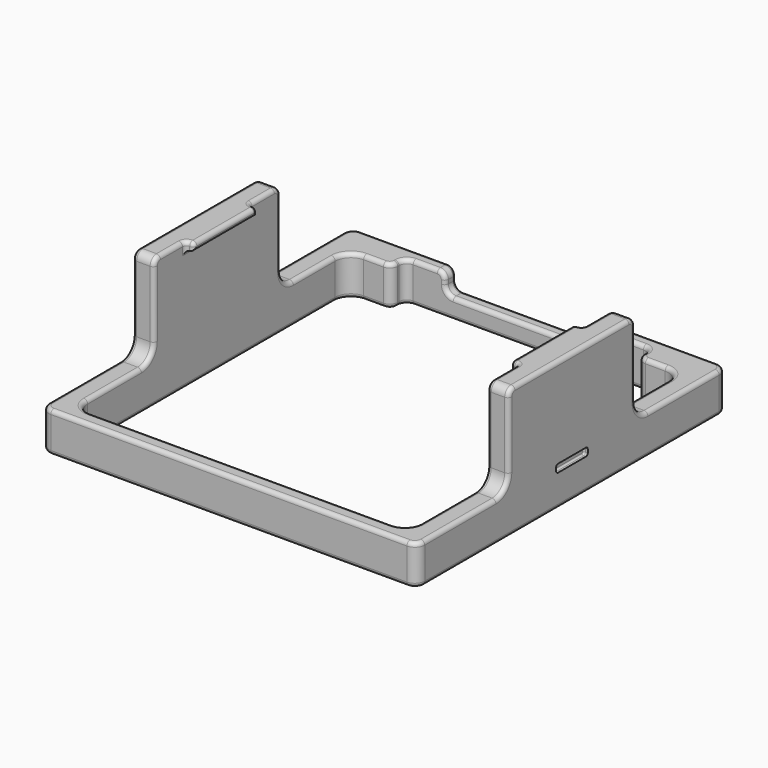
from build123d import *

# Parameters (mm, degrees)
F1_DEPTH      = 12.7
F2_W          = 53.34
F2_H          = 6.35
F3_DEPTH      = 4.318
F4_W          = 6.858
F4_H          = 50.8
F5_DEPTH      = 28.956
F7_W          = 25.4
F7_H          = 2.54
F8_DEPTH      = 2.54
F6_W          = 25.4
F6_H          = 2.54
F9_DEPTH      = 2.54
F10_R         = 5.08
F11_R         = 2.54
F12_R         = 1.26999
F13_R         = 2.54
F14_R         = 1.26999
F15_R         = 1.27
F16_W         = 12.7
F16_H         = 2.54
F18_DEPTH     = 1.27
F17_W         = 12.7
F17_H         = 2.54
F19_DEPTH     = 1.27
F20_R         = 0.508
F21_T1_DEPTH  = 1.27
F21_T3_DEPTH  = 1.27
F21_T6_ANGLE  = 90
F21_T8_ANGLE  = 90
F21_T10_ANGLE = 90
F21_T12_ANGLE = 90
F21_T14_ANGLE = 90
F21_T16_ANGLE = 90
F21_T18_ANGLE = 90
F21_T20_ANGLE = 90


# Not quite as in the source:
# - a fillet or chamfer that OpenCascade refuses, or shapes differently, is made with other operations: its cross-section is extruded or revolved along the edge and cut away or added
# - a fillet or chamfer is up to 0.001 mm smaller than in the source, because OpenCascade refuses the exact size


with BuildPart() as f1:
    # F0 (on Top) → F1 (new body)
    with BuildSketch(Plane.XY):
        with BuildLine():
            ThreePointArc((-60.325, -59.055), (-59.3950640303, -61.3000640303), (-57.15, -62.23))
            Line((-57.15, -62.23), (57.15, -62.23))
            ThreePointArc((57.15, -62.23), (59.3950640303, -61.3000640303), (60.325, -59.055))
            Line((60.325, -59.055), (60.325, 59.055))
            ThreePointArc((60.325, 59.055), (59.3950640303, 61.3000640303), (57.15, 62.23))
            Line((57.15, 62.23), (-57.15, 62.23))
            ThreePointArc((-57.15, 62.23), (-59.3950640303, 61.3000640303), (-60.325, 59.055))
            Line((-60.325, 59.055), (-60.325, -59.055))
        make_face()
        with BuildLine():
            Line((39.497, 52.324), (48.387, 52.324))
            ThreePointArc((48.387, 52.324), (51.9791024484, 50.8361024484), (53.467, 47.244))
            Line((53.467, 47.244), (53.467, -52.07))
            ThreePointArc((53.467, -52.07), (51.9791024484, -55.6621024484), (48.387, -57.15))
            Line((48.387, -57.15), (-48.387, -57.15))
            ThreePointArc((-48.387, -57.15), (-51.9791024484, -55.6621024484), (-53.467, -52.07))
            Line((-53.467, -52.07), (-53.467, 47.244))
            ThreePointArc((-53.467, 47.244), (-51.9791024484, 50.8361024484), (-48.387, 52.324))
            Line((-48.387, 52.324), (-39.497, 52.324))
            Line((-39.497, 52.324), (-39.497, 57.912))
            Line((-39.497, 57.912), (39.497, 57.912))
            Line((39.497, 57.912), (39.497, 52.324))
        make_face(mode=Mode.SUBTRACT)
    extrude(amount=F1_DEPTH)

    # F2 (on face) → F3 (cut, through all)
    with BuildSketch(Plane(origin=(0, 62.23, 0), x_dir=(-1, 0, 0), z_dir=(0, 1, 0))):
        with Locations((0, 9.525)):
            Rectangle(F2_W, F2_H)
    extrude(amount=-F3_DEPTH, mode=Mode.SUBTRACT)

    # F4 (on face) → F5 (join)
    with BuildSketch(Plane.XY.offset(12.7)):
        with Locations((56.896, 0)):
            Rectangle(F4_W, F4_H)
        with Locations((-56.896, 0)):
            Rectangle(F4_W, F4_H)
    extrude(amount=F5_DEPTH)

    # F7 (on face) → F8 (join)
    with BuildSketch(Plane(origin=(53.467, 0, 0), x_dir=(0, -1, 0), z_dir=(-1, 0, 0))):
        with Locations((0, 40.386)):
            Rectangle(F7_W, F7_H)
    extrude(amount=F8_DEPTH)

    # F6 (on face) → F9 (join)
    with BuildSketch(Plane.YZ.offset(-53.467)):
        with Locations((0, 40.386)):
            Rectangle(F6_W, F6_H)
    extrude(amount=F9_DEPTH)

    # F10
    f10_edges = [f1.edges().sort_by_distance(p)[0] for p in [
        (56.896, 25.4, 12.7),
        (-56.896, 25.4, 12.7),
        (56.896, -25.4, 12.7),
        (-56.896, -25.4, 12.7),
    ]]
    fillet(f10_edges, radius=F10_R)

    # F11
    f11_edges = [f1.edges().sort_by_distance(p)[0] for p in [
        (-56.896, -25.4, 41.656),
        (-56.896, 25.4, 41.656),
        (56.896, -25.4, 41.656),
        (56.896, 25.4, 41.656),
    ]]
    fillet(f11_edges, radius=F11_R)

    # F12 (radius 1.27 in the source; OpenCascade refuses exactly that, so slightly less here)
    f12_edges = [f1.edges().sort_by_distance(p)[0] for p in [
        (-50.927, -12.7, 40.386),
        (-50.927, 12.7, 40.386),
        (50.927, 12.7, 40.386),
        (50.927, -12.7, 40.386),
        (53.467, 0, 39.116),
        (-53.467, 0, 39.116),
        (-53.467, 12.7, 40.386),
        (53.467, 12.7, 40.386),
        (53.467, -12.7, 40.386),
        (-53.467, -12.7, 40.386),
        (50.927, 0, 39.116),
        (-50.927, 0, 39.116),
    ]]
    fillet(f12_edges, radius=F12_R)

    # F13
    f13_edges = [f1.edges().sort_by_distance(p)[0] for p in [
        (-39.497, 52.324, 6.35),
        (-26.67, 60.071, 12.7),
        (26.67, 60.071, 12.7),
        (39.497, 52.324, 6.35),
        (-39.497, 57.912, 6.35),
        (39.497, 57.912, 6.35),
        (26.67, 60.071, 6.35),
        (-26.67, 60.071, 6.35),
    ]]
    fillet(f13_edges, radius=F13_R)

    # F14 (radius 1.27 in the source; OpenCascade refuses exactly that, so slightly less here)
    f14_edges = [f1.edges().sort_by_distance(p)[0] for p in [
        (-53.467, 38.862, 12.7),
        (-51.979102, 50.836102, 12.7),
        (60.325, 44.7675, 12.7),
        (-43.18, 62.23, 12.7),
        (43.18, 62.23, 12.7),
        (59.395064, 61.300064, 12.7),
        (-59.395064, 61.300064, 12.7),
        (-60.325, 44.7675, 12.7),
        (60.325, 0, 0),
        (59.395064, 61.300064, 0),
    ]]
    fillet(f14_edges, radius=F14_R)

    # F15
    f15_edges = [f1.edges().sort_by_distance(p)[0] for p in [
        (-45.212, 52.324, 0),
        (-40.240949, 53.067949, 0),
    ]]
    fillet(f15_edges, radius=F15_R)

    # F16 (on face) → F18 (cut)
    with BuildSketch(Plane(origin=(-60.325, 0, 0), x_dir=(0, -1, 0), z_dir=(-1, 0, 0))):
        with Locations((0, 11.43)):
            Rectangle(F16_W, F16_H)
    extrude(amount=-F18_DEPTH, mode=Mode.SUBTRACT)

    # F17 (on face) → F19 (cut)
    with BuildSketch(Plane.YZ.offset(60.325)):
        with Locations((0, 11.43)):
            Rectangle(F17_W, F17_H)
    extrude(amount=-F19_DEPTH, mode=Mode.SUBTRACT)

    # F20
    f20_edges = [f1.edges().sort_by_distance(p)[0] for p in [
        (-59.055, 0, 10.16),
        (-59.055, 6.35, 11.43),
        (-59.055, 0, 12.7),
        (-59.055, -6.35, 11.43),
        (59.055, 0, 12.7),
        (59.055, -6.35, 11.43),
        (59.055, 0, 10.16),
        (59.055, 6.35, 11.43),
    ]]
    fillet(f20_edges, radius=F20_R)

    # F21: fillet of radius 0.762 on 8 edges, made by hand

    # F21_s2 → F21_t1 (join)
    with BuildSketch(Plane.YZ.offset(59.055)):
        with BuildLine():
            ThreePointArc((-5.588, 10.16), (-6.1268153673, 10.3831846327), (-6.35, 10.922))
            Line((-6.35, 10.922), (-6.35, 10.16))
            Line((-6.35, 10.16), (-5.588, 10.16))
        make_face()
        with BuildLine():
            ThreePointArc((-5.588, 12.7), (-6.1268153673, 12.4768153673), (-6.35, 11.938))
            Line((-6.35, 11.938), (-6.35, 12.7))
            Line((-6.35, 12.7), (-5.588, 12.7))
        make_face()
        with BuildLine():
            ThreePointArc((6.35, 11.938), (6.1268153673, 12.4768153673), (5.588, 12.7))
            Line((5.588, 12.7), (6.35, 12.7))
            Line((6.35, 12.7), (6.35, 11.938))
        make_face()
        with BuildLine():
            ThreePointArc((6.35, 10.922), (6.1268153673, 10.3831846327), (5.588, 10.16))
            Line((5.588, 10.16), (6.35, 10.16))
            Line((6.35, 10.16), (6.35, 10.922))
        make_face()
    extrude(amount=F21_T1_DEPTH)

    # F21_s4 → F21_t3 (join)
    with BuildSketch(Plane.YZ.offset(-60.325)):
        with BuildLine():
            ThreePointArc((-6.35, 10.922), (-6.1268153673, 10.3831846327), (-5.588, 10.16))
            Line((-5.588, 10.16), (-6.35, 10.16))
            Line((-6.35, 10.16), (-6.35, 10.922))
        make_face()
        with BuildLine():
            ThreePointArc((-6.35, 11.938), (-6.1268153673, 12.4768153673), (-5.588, 12.7))
            Line((-5.588, 12.7), (-6.35, 12.7))
            Line((-6.35, 12.7), (-6.35, 11.938))
        make_face()
        with BuildLine():
            ThreePointArc((5.588, 10.16), (6.1268153673, 10.3831846327), (6.35, 10.922))
            Line((6.35, 10.922), (6.35, 10.16))
            Line((6.35, 10.16), (5.588, 10.16))
        make_face()
        with BuildLine():
            ThreePointArc((6.35, 11.938), (6.1268153673, 12.4768153673), (5.588, 12.7))
            Line((5.588, 12.7), (6.35, 12.7))
            Line((6.35, 12.7), (6.35, 11.938))
        make_face()
    extrude(amount=F21_T3_DEPTH)

    # F21_s5 → F21_t6 (revolve)
    with BuildSketch(Plane.XY.offset(11.938)):
        with BuildLine():
            ThreePointArc((-59.055, 5.842), (-59.2037897552, 6.2012102448), (-59.563, 6.35))
            Line((-59.563, 6.35), (-59.055, 6.35))
            Line((-59.055, 6.35), (-59.055, 5.842))
        make_face()
    revolve(axis=Axis((-59.055, 5.588, 11.938), (1, 0, 0)), revolution_arc=F21_T6_ANGLE)

    # F21_s7 → F21_t8 (revolve)
    with BuildSketch(Plane.XZ.offset(-5.588)):
        with BuildLine():
            ThreePointArc((-59.055, 10.668), (-59.2037897552, 10.3087897552), (-59.563, 10.16))
            Line((-59.563, 10.16), (-59.055, 10.16))
            Line((-59.055, 10.16), (-59.055, 10.668))
        make_face()
    revolve(axis=Axis((-59.055, 5.588, 10.922), (1, 0, 0)), revolution_arc=F21_T8_ANGLE)

    # F21_s9 → F21_t10 (revolve)
    with BuildSketch(Plane.XZ.offset(5.588)):
        with BuildLine():
            ThreePointArc((-59.055, 12.192), (-59.2037897552, 12.5512102448), (-59.563, 12.7))
            Line((-59.563, 12.7), (-59.055, 12.7))
            Line((-59.055, 12.7), (-59.055, 12.192))
        make_face()
    revolve(axis=Axis((-59.055, -5.588, 11.938), (1, 0, 0)), revolution_arc=F21_T10_ANGLE)

    # F21_s11 → F21_t12 (revolve)
    with BuildSketch(Plane.XY.offset(10.922)):
        with BuildLine():
            ThreePointArc((-59.055, -5.842), (-59.2037897552, -6.2012102448), (-59.563, -6.35))
            Line((-59.563, -6.35), (-59.055, -6.35))
            Line((-59.055, -6.35), (-59.055, -5.842))
        make_face()
    revolve(axis=Axis((-59.055, -5.588, 10.922), (1, 0, 0)), revolution_arc=F21_T12_ANGLE)

    # F21_s13 → F21_t14 (revolve)
    with BuildSketch(Plane.XY.offset(10.922)):
        with BuildLine():
            ThreePointArc((59.055, 5.842), (59.2037897552, 6.2012102448), (59.563, 6.35))
            Line((59.563, 6.35), (59.055, 6.35))
            Line((59.055, 6.35), (59.055, 5.842))
        make_face()
    revolve(axis=Axis((59.055, 5.588, 10.922), (-1, 0, 0)), revolution_arc=F21_T14_ANGLE)

    # F21_s15 → F21_t16 (revolve)
    with BuildSketch(Plane.XZ.offset(-5.588)):
        with BuildLine():
            ThreePointArc((59.055, 12.192), (59.2037897552, 12.5512102448), (59.563, 12.7))
            Line((59.563, 12.7), (59.055, 12.7))
            Line((59.055, 12.7), (59.055, 12.192))
        make_face()
    revolve(axis=Axis((59.055, 5.588, 11.938), (-1, 0, 0)), revolution_arc=F21_T16_ANGLE)

    # F21_s17 → F21_t18 (revolve)
    with BuildSketch(Plane.XY.offset(11.938)):
        with BuildLine():
            ThreePointArc((59.055, -5.842), (59.2037897552, -6.2012102448), (59.563, -6.35))
            Line((59.563, -6.35), (59.055, -6.35))
            Line((59.055, -6.35), (59.055, -5.842))
        make_face()
    revolve(axis=Axis((59.055, -5.588, 11.938), (-1, 0, 0)), revolution_arc=F21_T18_ANGLE)

    # F21_s19 → F21_t20 (revolve)
    with BuildSketch(Plane.XZ.offset(5.588)):
        with BuildLine():
            ThreePointArc((59.055, 10.668), (59.2037897552, 10.3087897552), (59.563, 10.16))
            Line((59.563, 10.16), (59.055, 10.16))
            Line((59.055, 10.16), (59.055, 10.668))
        make_face()
    revolve(axis=Axis((59.055, -5.588, 10.922), (-1, 0, 0)), revolution_arc=F21_T20_ANGLE)


solid = f1.part
